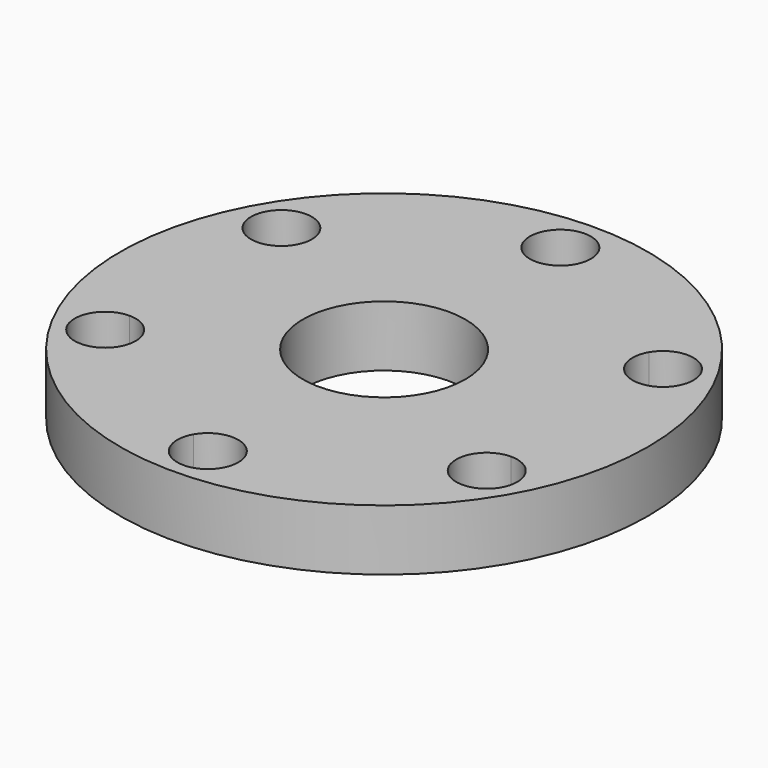
from build123d import *

# Parameters (mm, degrees)
F0_R     = 41.2696821878
F0_R_2   = 12.7004431624
F1_DEPTH = 9.525


# Not quite as in the source:
# - a feature names something its author has since deleted; it is built from what else it names


with BuildPart() as f1:
    # F0 (on Top) → F1 (new body)
    with BuildSketch(Plane.XY):
        Circle(F0_R)
        with BuildLine():
            ThreePointArc((34.593341478, 17.2228345975), (33.1984325721, 13.8552265986), (29.8308245732, 12.4603176927))
            Line((29.8308245732, 12.4603176927), (29.8308245732, -12.4556027445))
            ThreePointArc((29.8308245732, -12.4556027445), (33.201766544, -13.8518926268), (34.5980564262, -17.2228345975))
            ThreePointArc((34.5980564262, -17.2228345975), (31.0646749692, -21.8276269642), (25.7022806828, -19.606450524))
            Line((25.7022806828, -19.606450524), (4.1271236512, -32.062873244))
            ThreePointArc((4.1271236512, -32.062873244), (4.6032082956, -33.2122432496), (4.7655919019, -34.445669195))
            ThreePointArc((4.7655919019, -34.445669195), (-1.2334259454, -39.0488774906), (-4.1271236512, -32.062873244))
            Line((-4.1271236512, -32.062873244), (-25.7068508494, -19.6038119371))
            ThreePointArc((-25.7068508494, -19.6038119371), (-33.9547982971, -19.6038119371), (-29.8308245732, -12.4608799183))
            Line((-29.8308245732, -12.4608799183), (-29.8308245732, 12.464098707))
            ThreePointArc((-29.8308245732, 12.464098707), (-33.9520107443, 19.6022025428), (-25.7096384021, 19.6022025428))
            Line((-25.7096384021, 19.6022025428), (-4.1283119696, 32.062187168))
            ThreePointArc((-4.1283119696, 32.062187168), (-1.2337810845, 39.0502028877), (4.766964054, 34.445669195))
            ThreePointArc((4.766964054, 34.445669195), (4.6045336927, 33.2118881105), (4.1283119696, 32.062187168))
            Line((4.1283119696, 32.062187168), (25.7063639477, 19.6040930499))
            ThreePointArc((25.7063639477, 19.6040930499), (31.0634546508, 21.823072674), (34.593341478, 17.2228345975))
        make_face(mode=Mode.SUBTRACT)
        with BuildLine():
            Line((29.8308245732, -12.4556027445), (29.8308245732, 12.4603176927))
            ThreePointArc((29.8308245732, 12.4603176927), (25.7063639477, 14.8415761451), (25.7063639477, 19.6040930499))
            Line((25.7063639477, 19.6040930499), (4.1283119696, 32.062187168))
            ThreePointArc((4.1283119696, 32.062187168), (0, 29.6787051411), (-4.1283119696, 32.062187168))
            Line((-4.1283119696, 32.062187168), (-25.7096384021, 19.6022025428))
            ThreePointArc((-25.7096384021, 19.6022025428), (-25.2342386761, 18.4544860766), (-25.0720886827, 17.2228345975))
            ThreePointArc((-25.0720886827, 17.2228345975), (-26.4658901552, 13.8579001794), (-29.8308245732, 12.464098707))
            Line((-29.8308245732, 12.464098707), (-29.8308245732, -12.4608799183))
            ThreePointArc((-29.8308245732, -12.4608799183), (-26.4636141278, -13.8556241521), (-25.068869894, -17.2228345975))
            ThreePointArc((-25.068869894, -17.2228345975), (-25.231129565, -18.4553191604), (-25.7068508494, -19.6038119371))
            Line((-25.7068508494, -19.6038119371), (-4.1271236512, -32.062873244))
            ThreePointArc((-4.1271236512, -32.062873244), (0, -29.6800772931), (4.1271236512, -32.062873244))
            Line((4.1271236512, -32.062873244), (25.7022806828, -19.606450524))
            ThreePointArc((25.7022806828, -19.606450524), (25.7022806828, -14.839218671), (29.8308245732, -12.4556027445))
        make_face()
        Circle(F0_R_2, mode=Mode.SUBTRACT)
    extrude(amount=F1_DEPTH)


solid = f1.part
